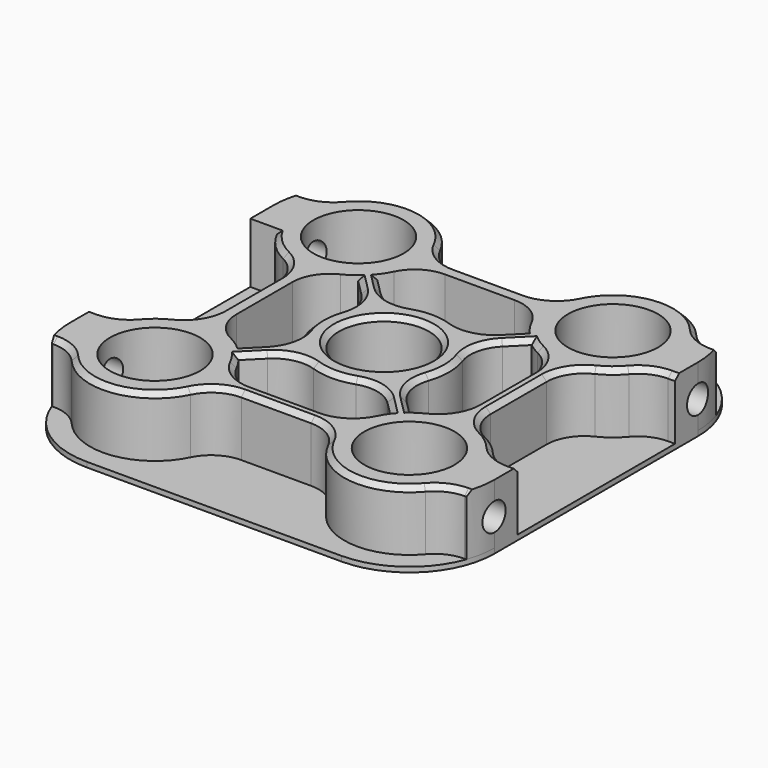
from build123d import *

# Parameters (mm, degrees)
F2_DEPTH  = 1
F0_R      = 9
F3_DEPTH  = 25
F4_R      = 9
F4_R_2    = 13
F6_DEPTH  = 12
F7_DEPTH  = 12
F9_R      = 2.7625
F12_DEPTH = 20
F11_R     = 2.7625
F13_DEPTH = 15
F16_DEPTH = 12
F17_DEPTH = 25
F14_R     = 5
F18_DEPTH = 25
F19_R     = 7.5
F20_SIZE  = 1


with BuildPart() as f2:
    # F1 (on Top) → F2 (new body)
    with BuildSketch(Plane.XY):
        with BuildLine():
            Line((-25.4, -42.4), (25.4, -42.4))
            ThreePointArc((25.4, -42.4), (37.4208152802, -37.4208152802), (42.4, -25.4))
            Line((42.4, -25.4), (42.4, 25.4))
            ThreePointArc((42.4, 25.4), (37.4208152802, 37.4208152802), (25.4, 42.4))
            Line((25.4, 42.4), (-25.4, 42.4))
            ThreePointArc((-25.4, 42.4), (-37.4208152802, 37.4208152802), (-42.4, 25.4))
            Line((-42.4, 25.4), (-42.4, -25.4))
            ThreePointArc((-42.4, -25.4), (-37.4208152802, -37.4208152802), (-25.4, -42.4))
        make_face()
    extrude(amount=F2_DEPTH)

    # F0 (on Top) → F3 (cut)
    with BuildSketch(Plane.XY):
        with Locations((-25.4, 25.4)):
            Circle(F0_R)
        with Locations((25.4, 25.4)):
            Circle(F0_R)
        with Locations((25.4, -25.4)):
            Circle(F0_R)
        with Locations((-25.4, -25.4)):
            Circle(F0_R)
        Circle(F0_R)
    extrude(amount=F3_DEPTH, mode=Mode.SUBTRACT)

    # F4 (on face) → F6 (join)
    with BuildSketch(Plane.XY.offset(1)):
        with BuildLine():
            Line((12.4868284299, 26.9), (-12.4868284299, 26.9))
            ThreePointArc((-12.4868284299, 26.9), (-34.5923881554, 34.5923881554), (-26.9, 12.4868284299))
            Line((-26.9, 12.4868284299), (-26.9, -12.4868284299))
            ThreePointArc((-26.9, -12.4868284299), (-34.5923881554, -34.5923881554), (-12.4868284299, -26.9))
            Line((-12.4868284299, -26.9), (12.4868284299, -26.9))
            ThreePointArc((12.4868284299, -26.9), (34.5923881554, -34.5923881554), (26.9, -12.4868284299))
            Line((26.9, -12.4868284299), (26.9, 12.4868284299))
            ThreePointArc((26.9, 12.4868284299), (34.5923881554, 34.5923881554), (12.4868284299, 26.9))
        make_face()
        with Locations((-25.4, -25.4)):
            Circle(F4_R, mode=Mode.SUBTRACT)
        with Locations((25.4, -25.4)):
            Circle(F4_R, mode=Mode.SUBTRACT)
        with Locations((-25.4, 25.4)):
            Circle(F4_R, mode=Mode.SUBTRACT)
        with BuildLine():
            Line((-12.4868284299, 23.9), (12.4868284299, 23.9))
            ThreePointArc((12.4868284299, 23.9), (16.2076118446, 16.2076118446), (23.9, 12.4868284299))
            Line((23.9, 12.4868284299), (23.9, -12.4868284299))
            ThreePointArc((23.9, -12.4868284299), (16.2076118446, -16.2076118446), (12.4868284299, -23.9))
            Line((12.4868284299, -23.9), (-12.4868284299, -23.9))
            ThreePointArc((-12.4868284299, -23.9), (-16.2076118446, -16.2076118446), (-23.9, -12.4868284299))
            Line((-23.9, -12.4868284299), (-23.9, 12.4868284299))
            ThreePointArc((-23.9, 12.4868284299), (-16.2076118446, 16.2076118446), (-12.4868284299, 23.9))
        make_face(mode=Mode.SUBTRACT)
        with Locations((25.4, 25.4)):
            Circle(F4_R, mode=Mode.SUBTRACT)
        Circle(F4_R_2)
        Circle(F4_R, mode=Mode.SUBTRACT)
    extrude(amount=F6_DEPTH)

    # F5 (on face) → F7 (join, through all)
    with BuildSketch(Plane.XY.offset(1)):
        with BuildLine():
            Line((-42.4, -19.6375), (-42.4, -25.4))
            ThreePointArc((-42.4, -25.4), (-42.1464970153, -28.3248654184), (-41.393548504, -31.1625))
            Line((-41.393548504, -31.1625), (-37.0530508344, -31.1625))
            ThreePointArc((-37.0530508344, -31.1625), (-38.4, -25.4), (-37.0530508344, -19.6375))
            Line((-37.0530508344, -19.6375), (-42.4, -19.6375))
        make_face()
        with BuildLine():
            ThreePointArc((41.393548504, -31.1625), (42.1464970153, -28.3248654184), (42.4, -25.4))
            Line((42.4, -25.4), (42.4, -19.6375))
            Line((42.4, -19.6375), (37.0530508344, -19.6375))
            ThreePointArc((37.0530508344, -19.6375), (38.4, -25.4), (37.0530508344, -31.1625))
            Line((37.0530508344, -31.1625), (41.393548504, -31.1625))
        make_face()
        with BuildLine():
            Line((-37.0530508344, 31.1625), (-41.393548504, 31.1625))
            ThreePointArc((-41.393548504, 31.1625), (-42.1464970153, 28.3248654184), (-42.4, 25.4))
            Line((-42.4, 25.4), (-42.4, 19.6375))
            Line((-42.4, 19.6375), (-37.0530508344, 19.6375))
            ThreePointArc((-37.0530508344, 19.6375), (-38.4, 25.4), (-37.0530508344, 31.1625))
        make_face()
        with BuildLine():
            Line((42.4, 19.6375), (42.4, 25.4))
            ThreePointArc((42.4, 25.4), (42.1464970153, 28.3248654184), (41.393548504, 31.1625))
            Line((41.393548504, 31.1625), (37.0530508344, 31.1625))
            ThreePointArc((37.0530508344, 31.1625), (38.4, 25.4), (37.0530508344, 19.6375))
            Line((37.0530508344, 19.6375), (42.4, 19.6375))
        make_face()
    extrude(amount=F7_DEPTH)

    # F9 (on offset) → F12 (cut)
    with BuildSketch(Plane(origin=(-42.4, 0, 0), x_dir=(0, -1, 0), z_dir=(-1, 0, 0))):
        with Locations((-25.4, 6.5)):
            Circle(F9_R)
        with Locations((25.4, 6.5)):
            Circle(F9_R)
    extrude(amount=-F12_DEPTH, mode=Mode.SUBTRACT)

    # F11 (on offset) → F13 (cut)
    with BuildSketch(Plane.YZ.offset(42.4)):
        with Locations((-25.4, 6.5)):
            Circle(F11_R)
        with Locations((25.4, 6.5)):
            Circle(F11_R)
    extrude(amount=-F13_DEPTH, mode=Mode.SUBTRACT)

    # F15 (on face) → F16 (join, through all)
    with BuildSketch(Plane.XY.offset(1)):
        with BuildLine():
            Line((15.2083486443, 17.3296689879), (8.0703310121, 10.1916513557))
            ThreePointArc((8.0703310121, 10.1916513557), (9.1923881554, 9.1923881554), (10.1916513557, 8.0703310121))
            Line((10.1916513557, 8.0703310121), (17.3296689879, 15.2083486443))
            ThreePointArc((17.3296689879, 15.2083486443), (16.2076118446, 16.2076118446), (15.2083486443, 17.3296689879))
        make_face()
        with BuildLine():
            Line((-17.3285065247, 15.2092692569), (-10.1925686307, 8.0691724922))
            ThreePointArc((-10.1925686307, 8.0691724922), (-9.1929105822, 9.191865699), (-8.0703310121, 10.1916513557))
            Line((-8.0703310121, 10.1916513557), (-15.2083486443, 17.3296689879))
            ThreePointArc((-15.2083486443, 17.3296689879), (-16.2070875924, 16.2081361267), (-17.3285065247, 15.2092692569))
        make_face()
        with BuildLine():
            Line((-10.1916513557, -8.0703310121), (-17.3296689879, -15.2083486443))
            ThreePointArc((-17.3296689879, -15.2083486443), (-16.2076118446, -16.2076118446), (-15.2083486443, -17.3296689879))
            Line((-15.2083486443, -17.3296689879), (-8.0703310121, -10.1916513557))
            ThreePointArc((-8.0703310121, -10.1916513557), (-9.1923881554, -9.1923881554), (-10.1916513557, -8.0703310121))
        make_face()
        with BuildLine():
            ThreePointArc((10.1916513557, -8.0703310121), (9.1919644172, -9.1928118741), (8.0693913978, -10.1923953254))
            Line((8.0693913978, -10.1923953254), (15.2090948081, -17.3287267813))
            ThreePointArc((15.2090948081, -17.3287267813), (16.2080367829, -16.2071869259), (17.3296689879, -15.2083486443))
            Line((17.3296689879, -15.2083486443), (10.1916513557, -8.0703310121))
        make_face()
    extrude(amount=F16_DEPTH)

    # F17 (cut): faces of the model
    f17_faces = [f2.faces().sort_by_distance(p)[0] for p in [
        (4.64667e-05, -18.0222040424, 1),
        (-18.0222146098, 5.74972e-05, 1),
        (0, 18.0221584642, 1),
        (18.0221584642, 0, 1),
    ]]
    extrude(f17_faces, amount=-F17_DEPTH, mode=Mode.SUBTRACT)

    # F14 (on face) → F18 (cut)
    with BuildSketch(Plane(origin=(0, 0, 0), x_dir=(1, 0, 0), z_dir=(0, 0, -1))):
        with Locations((18.5, 0)):
            Circle(F14_R)
        with Locations((0, 18.5)):
            Circle(F14_R)
        with Locations((-18.5, 0)):
            Circle(F14_R)
        with Locations((0, -18.5)):
            Circle(F14_R)
    extrude(amount=-F18_DEPTH, mode=Mode.SUBTRACT)

    # F19
    f19_edges = [f2.edges().sort_by_distance(p)[0] for p in [
        (26.9, 12.486828, 7),
        (26.9, -12.486828, 7),
        (-12.486828, -23.9, 6.5),
        (-23.9, -12.486828, 6.5),
        (-23.9, 12.486828, 6.5),
        (-12.486828, 23.9, 6.5),
        (12.486828, -23.9, 6.5),
        (23.9, -12.486828, 6.5),
        (-12.486828, -26.9, 7),
        (12.486828, -26.9, 7),
        (-37.053051, -31.1625, 7),
        (37.053051, -31.1625, 7),
        (37.053051, -19.6375, 7),
        (37.053051, 19.6375, 7),
        (12.486828, 23.9, 6.5),
        (12.486828, 26.9, 7),
        (-37.053051, 31.1625, 7),
        (-12.486828, 26.9, 7),
        (37.053051, 31.1625, 7),
        (-26.9, 12.486828, 7),
        (-26.9, -12.486828, 7),
        (-37.053051, -19.6375, 7),
        (-10.192569, 8.069172, 6.5),
        (-10.191651, -8.070331, 6.5),
        (-8.070331, -10.191651, 6.5),
        (8.069391, -10.192395, 6.5),
        (10.191651, -8.070331, 6.5),
        (10.191651, 8.070331, 6.5),
        (8.070331, 10.191651, 6.5),
        (-8.070331, 10.191651, 6.5),
        (23.9, 12.486828, 6.5),
    ]]
    fillet(f19_edges, radius=F19_R)

    # F20
    f20_edges = [f2.edges().sort_by_distance(p)[0] for p in [
        (37.880783, -18.943417, 13),
        (0, 26.9, 13),
        (-26.9, 0, 13),
        (0, -26.9, 13),
        (18.471088, -14.400447, 13),
        (14.400767, -18.470579, 13),
        (-9, 0, 13),
        (-13, 4.8e-05, 13),
        (-34.570623, 16.185898, 13),
        (-28.038195, 10.953342, 13),
        (-41.212721, 31.1625, 13),
        (-37.880783, 31.856583, 13),
        (-23.785247, 38.299324, 13),
        (-10.953342, 28.038195, 13),
        (10.953342, 28.038195, 13),
        (23.785247, 38.299324, 13),
        (37.880783, 31.856583, 13),
        (-28.038195, -10.953342, 13),
        (41.212721, 31.1625, 13),
        (-33.379397, -15.136997, 13),
        (-37.880783, -18.943417, 13),
        (-41.715947, -19.6375, 13),
        (41.715947, 19.6375, 13),
        (37.880783, 18.943417, 13),
        (33.379397, 15.136997, 13),
        (-41.212721, -31.1625, 13),
        (28.038195, 10.953342, 13),
        (-37.880783, -31.856583, 13),
        (26.9, 0, 13),
        (-23.785247, -38.299324, 13),
        (28.038195, -10.953342, 13),
        (-10.953342, -28.038195, 13),
        (33.379397, -15.136997, 13),
        (10.953342, -28.038195, 13),
        (41.715947, -19.6375, 13),
        (23.785247, -38.299324, 13),
        (37.880783, -31.856583, 13),
        (41.212721, -31.1625, 13),
        (-15.707173, -13.585852, 13),
        (-15.705795, 13.585612, 13),
        (-12.080816, -8.349844, 13),
        (-12.080514, 8.348896, 13),
        (-13.585852, 15.707173, 13),
        (-8.349844, 12.080816, 13),
        (0, 13, 13),
        (8.349844, 12.080816, 13),
        (13.585852, 15.707173, 13),
        (18.471088, 14.400447, 13),
        (22.761805, 10.953342, 13),
        (15.707173, 13.585852, 13),
        (23.9, 0, 13),
        (12.080816, 8.349844, 13),
        (22.761805, -10.953342, 13),
        (13, 0, 13),
        (12.080816, -8.349844, 13),
        (15.707173, -13.585852, 13),
        (10.953342, -22.761805, 13),
        (13.585657, -15.706056, 13),
        (0, -23.9, 13),
        (8.349075, -12.080571, 13),
        (-10.953342, -22.761805, 13),
        (3.9e-05, -13, 13),
        (-14.400447, -18.471088, 13),
        (-8.349844, -12.080816, 13),
        (-13.585852, -15.707173, 13),
    ]]
    chamfer(f20_edges, length=F20_SIZE)


solid = f2.part
